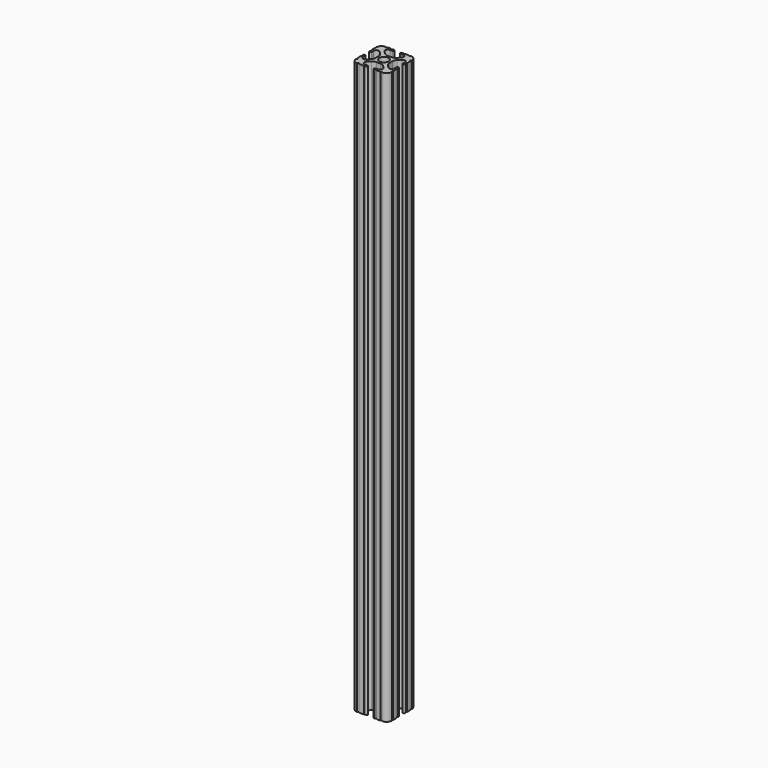
from build123d import *

# Parameters (mm, degrees)
F0_R     = 3.3625011168
F1_DEPTH = 406.4


# Not quite as in the source:
# - ends of sketch curves that miss each other by under 0.0002 mm in the source are joined


with BuildPart() as f1:
    # F0 (on Top) → F1 (new body)
    with BuildSketch(Plane.XY):
        with BuildLine():
            ThreePointArc((-8.5485764575, 18.7552378401), (-9.7846294165, 17.9293336576), (-11.2426532939, 17.6393146764))
            Line((-11.2426532939, 17.6393146764), (-14.1573467061, 17.6393146764))
            ThreePointArc((-14.1573467061, 17.6393146764), (-15.6153705835, 17.9293336576), (-16.8514235425, 18.7552378401))
            Line((-16.8514235425, 18.7552378401), (-18.696905198, 20.6007194956))
            ThreePointArc((-18.696905198, 20.6007194956), (-19.1098572893, 22.6767698525), (-17.3498667798, 23.8527579138))
            Line((-17.3498667798, 23.8527579138), (-15.6153705835, 23.8527579138))
            Line((-15.6153705835, 23.8527579138), (-15.5830195394, 23.8527579138))
            ThreePointArc((-15.5830195394, 23.8527579138), (-14.8254049311, 24.6263789569), (-15.5830195394, 25.4))
            Line((-15.5830195394, 25.4), (-15.6153705835, 25.4))
            Line((-15.6153705835, 25.4), (-16.2533409894, 25.4))
            ThreePointArc((-16.2533409894, 25.4), (-16.8016038846, 24.8587722652), (-17.3498667798, 25.4))
            Line((-17.3498667798, 25.4), (-20.4874817282, 25.4))
            ThreePointArc((-20.4874817282, 25.4), (-21.0387408641, 24.8487408595), (-21.5900000046, 25.4))
            ThreePointArc((-21.5900000046, 25.4), (-24.2840768363, 24.2840768363), (-25.4, 21.59))
            Line((-25.4, 21.59), (-25.4, 20.5047242343))
            Line((-25.4, 20.5047242343), (-25.4, 17.3498667798))
            ThreePointArc((-25.4, 17.3498667798), (-24.8441605755, 16.8026749055), (-25.4, 16.2554830313))
            Line((-25.4, 16.2554830313), (-25.4, 15.6153705835))
            ThreePointArc((-25.4, 15.6153705835), (-24.6263789569, 14.8595541131), (-23.8527579138, 15.6153705835))
            Line((-23.8527579138, 15.6153705835), (-23.8527579138, 17.3498667798))
            ThreePointArc((-23.8527579138, 17.3498667798), (-22.6767698525, 19.1098572893), (-20.6007194956, 18.696905198))
            Line((-20.6007194956, 18.696905198), (-18.7552378401, 16.8514235425))
            ThreePointArc((-18.7552378401, 16.8514235425), (-17.9293336576, 15.6153705835), (-17.6393146764, 14.1573467061))
            Line((-17.6393146764, 14.1573467061), (-17.6393146764, 11.2426532939))
            ThreePointArc((-17.6393146764, 11.2426532939), (-17.9293336576, 9.7846294165), (-18.7552378401, 8.5485764575))
            Line((-18.7552378401, 8.5485764575), (-20.6007194956, 6.703094802))
            ThreePointArc((-20.6007194956, 6.703094802), (-22.6767698525, 6.2901427107), (-23.8527579138, 8.0501332202))
            Line((-23.8527579138, 8.0501332202), (-23.8527579138, 9.7846294165))
            ThreePointArc((-23.8527579138, 9.7846294165), (-24.6263789569, 10.5582546272), (-25.4000041675, 9.7846294165))
            Line((-25.4000041675, 9.7846294165), (-25.4, 9.1492393985))
            ThreePointArc((-25.4, 9.1492393985), (-24.8993742936, 8.5996863094), (-25.4, 8.0501332202))
            Line((-25.4, 8.0501332202), (-25.4, 4.904538393))
            ThreePointArc((-25.4, 4.904538393), (-24.8462160257, 4.3572691965), (-25.4, 3.81))
            ThreePointArc((-25.4, 3.81), (-24.2840768363, 1.1159231637), (-21.59, 0))
            ThreePointArc((-21.59, 0), (-21.0408167821, 0.5548848314), (-20.4916335642, 0))
            Line((-20.4916335642, 0), (-16.7081691325, 0))
            ThreePointArc((-16.7081691325, 0), (-16.161769858, 0.5401345174), (-15.6153705835, 0))
            ThreePointArc((-15.6153705835, 0), (-14.8541835334, 0.7747), (-15.6153705835, 1.5494))
            Line((-15.6153705835, 1.5494), (-17.347708866, 1.5494))
            ThreePointArc((-17.347708866, 1.5494), (-19.1076993754, 2.7253880613), (-18.6947472842, 4.8014384182))
            Line((-18.6947472842, 4.8014384182), (-16.8514235425, 6.6447621599))
            ThreePointArc((-16.8514235425, 6.6447621599), (-15.6153705835, 7.4706663424), (-14.1573467061, 7.7606853236))
            Line((-14.1573467061, 7.7606853236), (-11.2426532939, 7.7606853236))
            ThreePointArc((-11.2426532939, 7.7606853236), (-9.7846294165, 7.4706663424), (-8.5485764575, 6.6447621599))
            Line((-8.5485764575, 6.6447621599), (-6.7052527158, 4.8014384182))
            ThreePointArc((-6.7052527158, 4.8014384182), (-6.2923006246, 2.7253880613), (-8.052291134, 1.5494))
            Line((-8.052291134, 1.5494), (-9.7846294165, 1.5494))
            ThreePointArc((-9.7846294165, 1.5494), (-10.4018355229, 0.7747), (-9.7846294165, 0))
            Line((-9.7846294165, 0), (-9.1528678313, 0))
            ThreePointArc((-9.1528678313, 0), (-8.6025794826, 0.5452621138), (-8.052291134, 0))
            Line((-8.052291134, 0), (-4.8988661729, 0))
            ThreePointArc((-4.8988661729, 0), (-4.3544330864, 0.5444330864), (-3.81, 0))
            ThreePointArc((-3.81, 0), (-1.1159231637, 1.1159231637), (0, 3.81))
            ThreePointArc((0, 3.81), (-0.5393803924, 4.3561), (0, 4.9022))
            Line((0, 4.9022), (0, 8.052291134))
            ThreePointArc((0, 8.052291134), (-0.5435172497, 8.6016602673), (0, 9.1510294005))
            Line((0, 9.1510294005), (0, 9.7846294165))
            ThreePointArc((0, 9.7846294165), (-0.7747, 10.5046907664), (-1.5494, 9.7846294165))
            Line((-1.5494, 9.7846294165), (-1.5494, 8.052291134))
            ThreePointArc((-1.5494, 8.052291134), (-2.7253880613, 6.2923006246), (-4.8014384182, 6.7052527158))
            Line((-4.8014384182, 6.7052527158), (-6.6447621599, 8.5485764575))
            ThreePointArc((-6.6447621599, 8.5485764575), (-7.4706663424, 9.7846294165), (-7.7606853236, 11.2426532939))
            Line((-7.7606853236, 11.2426532939), (-7.7606853236, 14.1573467061))
            ThreePointArc((-7.7606853236, 14.1573467061), (-7.4706663424, 15.6153705835), (-6.6447621599, 16.8514235425))
            Line((-6.6447621599, 16.8514235425), (-4.8014384182, 18.6947472842))
            ThreePointArc((-4.8014384182, 18.6947472842), (-2.7253880613, 19.1076993754), (-1.5494, 17.347708866))
            Line((-1.5494, 17.347708866), (-1.5494, 15.6153705835))
            ThreePointArc((-1.5494, 15.6153705835), (-0.7747, 14.8794054827), (0, 15.6153705835))
            Line((0, 15.6153705835), (0, 16.255508866))
            ThreePointArc((0, 16.255508866), (-0.5461, 16.801608866), (0, 17.347708866))
            Line((0, 17.347708866), (0, 20.4951651394))
            ThreePointArc((0, 20.4951651394), (-0.5510556267, 21.0425825697), (0, 21.59))
            ThreePointArc((0, 21.59), (-1.1159231637, 24.2840768363), (-3.81, 25.4))
            ThreePointArc((-3.81, 25.4), (-4.3653028659, 24.9036192847), (-4.9206057318, 25.4))
            Line((-4.9206057318, 25.4), (-8.0501332202, 25.4))
            ThreePointArc((-8.0501332202, 25.4), (-8.5963647474, 24.8594330871), (-9.1425962746, 25.4))
            Line((-9.1425962746, 25.4), (-9.7846294165, 25.4))
            Line((-9.7846294165, 25.4), (-9.856202747, 25.4))
            ThreePointArc((-9.856202747, 25.4), (-10.594864404, 24.6263789569), (-9.856202747, 23.8527579138))
            Line((-9.856202747, 23.8527579138), (-9.7846294165, 23.8527579138))
            Line((-9.7846294165, 23.8527579138), (-8.0501332202, 23.8527579138))
            ThreePointArc((-8.0501332202, 23.8527579138), (-6.2901427107, 22.6767698525), (-6.703094802, 20.6007194956))
            Line((-6.703094802, 20.6007194956), (-8.5485764575, 18.7552378401))
        make_face()
        with Locations((-12.7, 12.7)):
            Circle(F0_R, mode=Mode.SUBTRACT)
        with BuildLine():
            ThreePointArc((-9.856202747, 23.8527579138), (-9.8204160818, 23.8519306347), (-9.7846294165, 23.8527579138))
            Line((-9.7846294165, 23.8527579138), (-9.856202747, 23.8527579138))
        make_face()
        with BuildLine():
            Line((-15.5830195394, 23.8527579138), (-15.6153705835, 23.8527579138))
            ThreePointArc((-15.6153705835, 23.8527579138), (-15.5991950614, 23.8525888265), (-15.5830195394, 23.8527579138))
        make_face()
        with BuildLine():
            ThreePointArc((-9.7846294165, 25.4), (-9.8204160818, 25.4008272791), (-9.856202747, 25.4))
            Line((-9.856202747, 25.4), (-9.7846294165, 25.4))
        make_face()
        with BuildLine():
            Line((-15.6153705835, 25.4), (-15.5830195394, 25.4))
            ThreePointArc((-15.5830195394, 25.4), (-15.5991950614, 25.4001690873), (-15.6153705835, 25.4))
        make_face()
    extrude(amount=F1_DEPTH)


solid = f1.part
